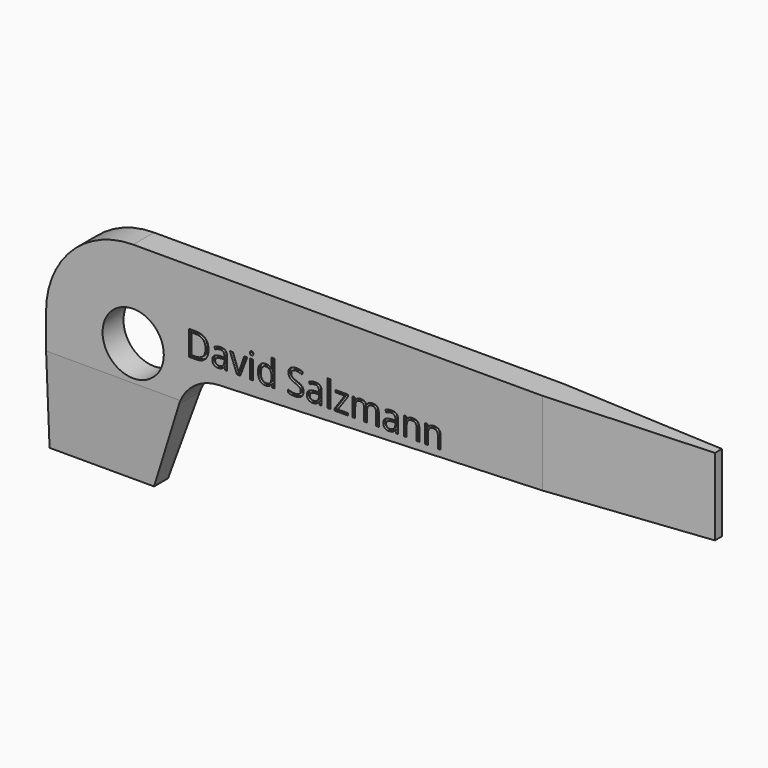
from build123d import *

# Parameters (mm, degrees)
F1_DEPTH     = 2.38125
F2_R         = 2.7915074899
F3_DEPTH     = 2.38225
F5_DEPTH     = 19.051
F7_DEPTH     = 60.326
F8_TEXT_SIZE = 3.1553942406
F9_DEPTH     = 0.2286


# Not quite as in the source:
# - Text() gives the source's letters only with a copy of the font that has no kerning and outlines rounded to 1/6400 em; it was checked with that copy


with BuildPart() as f1:
    # F0 (on Front) → F1 (new body)
    with BuildSketch(Plane.XZ):
        with BuildLine():
            Line((-11.4696488114, 8.8550521951), (-11.4696488114, -2.2574478049))
            Line((-11.4696488114, -2.2574478049), (-1.9446488114, -2.2574478049))
            Line((-1.9446488114, -2.2574478049), (0.6477159761, 5.3697186576))
            ThreePointArc((0.6477159761, 5.3697186576), (2.0327932341, 7.2740526768), (4.2530987567, 8.0583807037))
            Line((4.2530987567, 8.0583807037), (48.8553511886, 9.7707092584))
            Line((48.8553511886, 9.7707092584), (48.8553511886, 16.7925521951))
            Line((48.8553511886, 16.7925521951), (-3.5321488114, 16.7925521951))
            ThreePointArc((-3.5321488114, 16.7925521951), (-9.1448088871, 14.4677122708), (-11.4696488114, 8.8550521951))
        make_face()
    extrude(amount=F1_DEPTH)

    # F2 (on face) → F3 (cut, through all)
    with BuildSketch(Plane.XZ.offset(2.38125)):
        with Locations((-3.5321488114, 8.8550521951)):
            Circle(F2_R)
    extrude(amount=-F3_DEPTH, mode=Mode.SUBTRACT)

    # F4 (on face) → F5 (cut, through all)
    with BuildSketch(Plane.XY.offset(16.7925521951)):
        Polygon((48.8553511886, 0), (33.7741011886, 0), (48.8553511886, -0.79375), align=None)
        Polygon((48.8553511886, -1.5875), (33.7741011886, -2.38125), (48.8553511886, -2.38125), align=None)
    extrude(amount=-F5_DEPTH, mode=Mode.SUBTRACT)

    # F6 (on face) → F7 (cut, through all)
    with BuildSketch(Plane(origin=(-11.4696488114, 0, 0), x_dir=(0, -1, 0), z_dir=(-1, 0, 0))):
        Polygon((0.396875, -2.2574478049), (0, 5.6800521951), (0, -2.2574478049), align=None)
        Polygon((2.38125, -2.2574478049), (2.38125, 5.6800521951), (1.984375, -2.2574478049), align=None)
    extrude(amount=-F7_DEPTH, mode=Mode.SUBTRACT)

    # F8 (on face) → F9 (cut)
    with BuildSketch(Plane.XZ.offset(2.38125)):
        with Locations((1.2303511886, 9.4406683419)):
            Text('David Salzmann', F8_TEXT_SIZE, font='Open Sans', text_align=(TextAlign.LEFT, TextAlign.BOTTOM))
    extrude(amount=-F9_DEPTH, mode=Mode.SUBTRACT)


solid = f1.part
